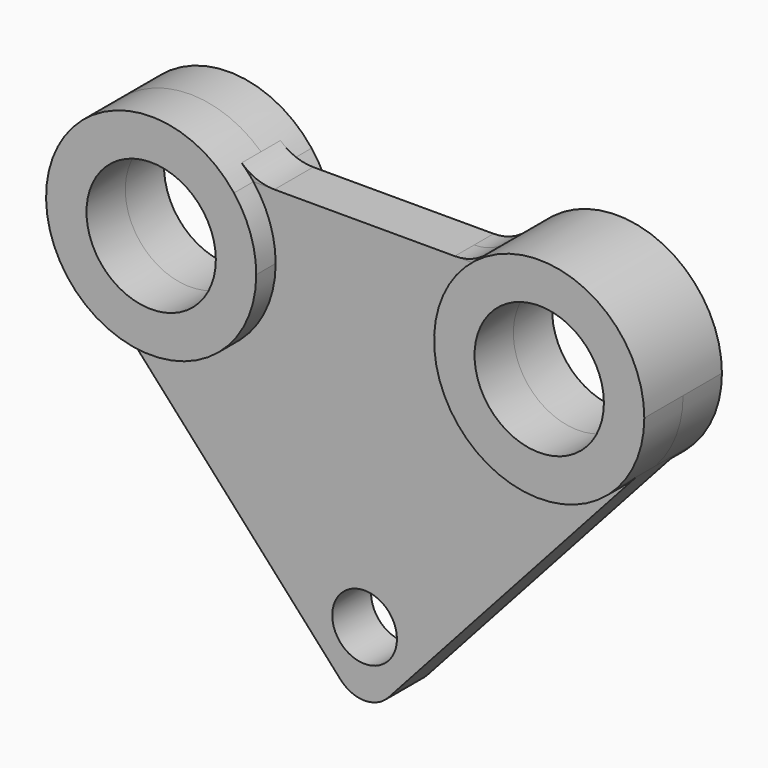
from build123d import *

# Parameters (mm, degrees)
F0_R        = 20
F1_DEPTH    = 15
F0_R_2      = 10
F2_DEPTH    = 7.5
F3_T1_DEPTH = 7.5
F3_T3_DEPTH = 7.5


# Not quite as in the source:
# - a fillet or chamfer that OpenCascade refuses, or shapes differently, is made with other operations: its cross-section is extruded or revolved along the edge and cut away or added


with BuildPart() as f1:
    # F0 (on Front) → F1 (new body, symmetric)
    with BuildSketch(Plane.XZ):
        with BuildLine():
            ThreePointArc((-24.128180818, -21.7733986877), (11.6637070311, -30.3349293438), (32.5, 0))
            ThreePointArc((32.5, 0), (30.7312117377, 10.5755673669), (25.6173769149, 20))
            ThreePointArc((25.6173769149, 20), (-20.899967362, 24.8885789925), (-24.128180818, -21.7733986877))
        make_face()
        Circle(F0_R, mode=Mode.SUBTRACT)
    extrude(amount=F1_DEPTH, both=True)



with BuildPart() as f1b:
    # F0 (on Front) → F1, piece 2 (new body, symmetric)
    with BuildSketch(Plane.XZ):
        with BuildLine():
            ThreePointArc((152.5, 0), (130.5755673669, 30.7312117377), (94.3826230851, 20))
            ThreePointArc((94.3826230851, 20), (99.100032638, -24.8885789925), (144.128180818, -21.7733986877))
            ThreePointArc((144.128180818, -21.7733986877), (150.3349293438, -11.6637070311), (152.5, 0))
        make_face()
        with Locations((120, 0)):
            Circle(F0_R, mode=Mode.SUBTRACT)
    extrude(amount=F1_DEPTH, both=True)


with BuildPart() as f1_1:
    add(f1.part)

    add(f1b.part)  # F2 merges F1b
    # F0 (on Front) → F2 (join, symmetric)
    with BuildSketch(Plane.XZ):
        with BuildLine():
            ThreePointArc((25.6173769149, 20), (30.7312117377, 10.5755673669), (32.5, 0))
            ThreePointArc((32.5, 0), (11.6637070311, -30.3349293438), (-24.128180818, -21.7733986877))
            Line((-24.128180818, -21.7733986877), (52.5759443637, -106.773036476))
            ThreePointArc((52.5759443637, -106.773036476), (60, -110.0735291875), (67.4240556363, -106.773036476))
            Line((67.4240556363, -106.773036476), (144.128180818, -21.7733986877))
            ThreePointArc((144.128180818, -21.7733986877), (99.100032638, -24.8885789925), (94.3826230851, 20))
            Line((94.3826230851, 20), (25.6173769149, 20))
        make_face()
        with Locations((60, -90.0735291875)):
            Circle(F0_R_2, mode=Mode.SUBTRACT)
    extrude(amount=F2_DEPTH, both=True)

    # F3: fillet of radius 15 on 4 edges, made by hand

    # F3_s2 → F3_t1 (join)
    with BuildSketch(Plane.XZ.offset(-7.5)):
        with BuildLine():
            ThreePointArc((32.1130814467, 20), (26.6720095708, 21.0216332556), (21.9721083582, 23.9473684211))
            ThreePointArc((21.9721083582, 23.9473684211), (23.8764571598, 22.0491449607), (25.6173769149, 20))
            Line((25.6173769149, 20), (32.1130814467, 20))
        make_face()
        with BuildLine():
            ThreePointArc((98.0278916418, 23.9473684211), (93.3279904292, 21.0216332556), (87.8869185533, 20))
            Line((87.8869185533, 20), (94.3826230851, 20))
            ThreePointArc((94.3826230851, 20), (96.1235428402, 22.0491449607), (98.0278916418, 23.9473684211))
        make_face()
    extrude(amount=F3_T1_DEPTH)

    # F3_s4 → F3_t3 (join)
    with BuildSketch(Plane.XZ):
        with BuildLine():
            ThreePointArc((32.1130814467, 20), (26.6720095708, 21.0216332556), (21.9721083582, 23.9473684211))
            ThreePointArc((21.9721083582, 23.9473684211), (23.8764571598, 22.0491449607), (25.6173769149, 20))
            Line((25.6173769149, 20), (32.1130814467, 20))
        make_face()
        with BuildLine():
            ThreePointArc((87.8869185533, 20), (93.3279904292, 21.0216332556), (98.0278916418, 23.9473684211))
            ThreePointArc((98.0278916418, 23.9473684211), (96.1235428402, 22.0491449607), (94.3826230851, 20))
            Line((94.3826230851, 20), (87.8869185533, 20))
        make_face()
    extrude(amount=F3_T3_DEPTH)


solid = f1_1.part
